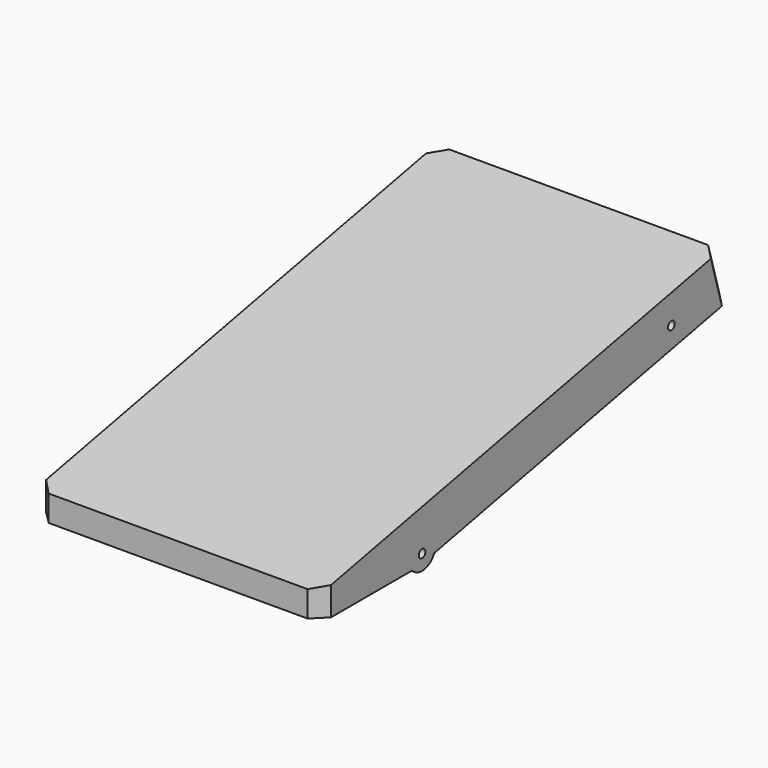
from build123d import *

# Parameters (mm, degrees)
F1_R         = 1.6
F2_DEPTH     = 110
F3_W         = 15
F3_H         = 15
F4_DEPTH     = 10.5
F5_R         = 1.6
F6_DEPTH     = 15
F7_T1_DEPTH  = 15
F9_DEPTH     = 5
F10_R        = 1.6
F11_DEPTH    = 110.001
F12_SIZE     = 5
F13_SIZE     = 5
F14_SIZE     = 5
F15_R        = 1.6
F16_DEPTH    = 15
F17_T1_DEPTH = 15


# Not quite as in the source:
# - a fillet or chamfer that OpenCascade refuses, or shapes differently, is made with other operations: its cross-section is extruded or revolved along the edge and cut away or added
# - an extrude ends at something that could not be found from the text; its depth is read off the source's solid


with BuildPart() as f2:
    # F1 (on Right) → F2 (new body)
    with BuildSketch(Plane.YZ):
        with BuildLine():
            Line((-97.5568636432, 0), (-53.34897794, 0))
            ThreePointArc((-53.34897794, 0), (-47.6134207396, -2.0300236301), (-42.7112703662, 1.5736597709))
            Line((-42.7112703662, 1.5736597709), (101.0891949998, 30.1261963412))
            Line((101.0891949998, 30.1261963412), (95.775378419, 48.3873994959))
            Line((95.775378419, 48.3873994959), (-97.5568636432, 10))
            Line((-97.5568636432, 10), (-97.5568636432, 0))
        make_face()
        with Locations((-48.5646284544, 3.8089532984)):
            Circle(F1_R, mode=Mode.SUBTRACT)
    extrude(amount=F2_DEPTH)

    # F3 (on Top) → F4 (cut, symmetric)
    with BuildSketch(Plane.XY):
        with Locations((22.5, -48.34897794)):
            Rectangle(F3_W, F3_H)
        with Locations((87.5, -47.7112703662)):
            Rectangle(F3_W, F3_H)
    extrude(amount=F4_DEPTH, both=True, mode=Mode.SUBTRACT)

    # F5 (on face) → F6 (cut, through all)
    with BuildSketch(Plane.YZ.offset(80)):
        with BuildLine():
            Line((-28.9665386081, -1.5009464696), (-35.5646284544, 3.8089532984))
            ThreePointArc((-35.5646284544, 3.8089532984), (-48.5646284544, 16.8089532984), (-61.5646284544, 3.8089532984))
            Line((-61.5646284544, 3.8089532984), (-67.6559507847, -1.5009464696))
            Line((-67.6559507847, -1.5009464696), (-44.5721596479, -13.8469105586))
            Line((-44.5721596479, -13.8469105586), (-28.9665386081, -1.5009464696))
        make_face()
        with Locations((-48.5646284544, 3.8089532984)):
            Circle(F5_R, mode=Mode.SUBTRACT)
    extrude(amount=F6_DEPTH, mode=Mode.SUBTRACT)

    # F7: chamfer of 5 on 1 edges, made by hand

    # F7_s2 → F7_t1 (cut)
    with BuildSketch(Plane.YZ.offset(80)):
        with BuildLine():
            Line((-64.7812034248, 0.9241461465), (-61.1056580828, 6.9991937656))
            Line((-61.1056580828, 6.9991937656), (-61.0083922357, 6.9759697482))
            ThreePointArc((-61.0083922357, 6.9759697482), (-61.3651603236, 5.4078228571), (-61.4646284544, 3.8089532984))
            Line((-61.4646284544, 3.8089532984), (-61.4989183361, 3.7335730599))
            ThreePointArc((-61.4989183361, 3.7335730599), (-63.1272340331, 2.3141451142), (-64.7154933066, 0.848765908))
            Line((-64.7154933066, 0.848765908), (-64.7812034248, 0.9241461465))
        make_face()
    extrude(amount=F7_T1_DEPTH, mode=Mode.SUBTRACT)

    # F8 (on offset) → F9 (cut, symmetric)
    with BuildSketch(Plane.YZ.offset(55)):
        with BuildLine():
            Line((77.775378419, 22.0739301294), (77.775378419, 32.4073002482))
            ThreePointArc((77.775378419, 32.4073002482), (71.775378419, 38.4073002482), (65.775378419, 32.4073002482))
            Line((65.775378419, 32.4073002482), (65.775378419, 22.0739301294))
            Line((65.775378419, 22.0739301294), (77.775378419, 22.0739301294))
        make_face()
    extrude(amount=F9_DEPTH, both=True, mode=Mode.SUBTRACT)

    # F10 (on face) → F11 (cut, through all)
    with BuildSketch(Plane.YZ.offset(110)):
        with Locations((71.775378419, 32.4073002482)):
            Circle(F10_R)
    extrude(amount=-F11_DEPTH, mode=Mode.SUBTRACT)

    # F12
    f12_edges = [f2.edges().sort_by_distance(p)[0] for p in [
        (55, 77.775378, 25.497083),
    ]]
    chamfer(f12_edges, length=F12_SIZE)

    # F13
    f13_edges = [f2.edges().sort_by_distance(p)[0] for p in [
        (55, 65.775378, 23.114404),
    ]]
    chamfer(f13_edges, length=F13_SIZE)

    # F14
    f14_edges = [f2.edges().sort_by_distance(p)[0] for p in [
        (0, 98.432287, 39.256798),
        (110, 98.432287, 39.256798),
        (110, -97.556864, 5),
        (0, -97.556864, 5),
    ]]
    chamfer(f14_edges, length=F14_SIZE)

    # F15 (on face) → F16 (cut, through all)
    with BuildSketch(Plane(origin=(30, 0, 0), x_dir=(0, -1, 0), z_dir=(-1, 0, 0))):
        with BuildLine():
            Line((68.1627183007, -1.5009464696), (61.5646284544, 3.8089532984))
            ThreePointArc((61.5646284544, 3.8089532984), (48.5646284544, 16.8089532984), (35.5646284544, 3.8089532984))
            Line((35.5646284544, 3.8089532984), (29.4733061241, -1.5009464696))
            Line((29.4733061241, -1.5009464696), (52.5570972608, -13.8469105586))
            Line((52.5570972608, -13.8469105586), (68.1627183007, -1.5009464696))
        make_face()
        with Locations((48.5646284544, 3.8089532984)):
            Circle(F15_R, mode=Mode.SUBTRACT)
    extrude(amount=F16_DEPTH, mode=Mode.SUBTRACT)

    # F17: chamfer of 5 on 1 edges, made by hand

    # F17_s2 → F17_t1 (cut)
    with BuildSketch(Plane.YZ.offset(15)):
        with BuildLine():
            Line((-64.9047662945, 1.0383670147), (-61.0901119265, 7.0462123799))
            Line((-61.0901119265, 7.0462123799), (-60.9929374028, 7.0226091613))
            ThreePointArc((-60.9929374028, 7.0226091613), (-61.3621185428, 5.4319897848), (-61.4646284544, 3.8089532984))
            Line((-61.4646284544, 3.8089532984), (-61.5019329447, 3.731047759))
            ThreePointArc((-61.5019329447, 3.731047759), (-63.1921659154, 2.3708104982), (-64.8420707848, 0.9604614753))
            Line((-64.8420707848, 0.9604614753), (-64.9047662945, 1.0383670147))
        make_face()
    extrude(amount=F17_T1_DEPTH, mode=Mode.SUBTRACT)


solid = f2.part
